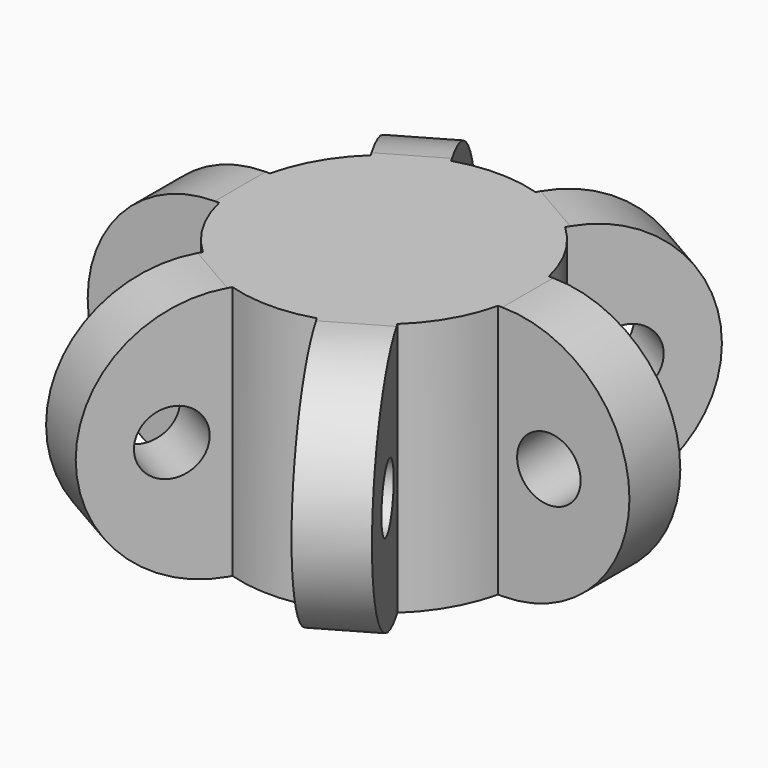
from build123d import *

# Parameters (mm, degrees)
F0_R            = 28.575
F1_DEPTH        = 50.8
F2_R            = 25.4
F3_DEPTH        = 25.4
F5_DEPTH        = 6.35
F5_DEPTH_BACK   = 6.35
F5_COPIES_COUNT = 6
F6_R            = 6.35
F7_DEPTH        = 25.4
F7_COPIES_COUNT = 6


# Not quite as in the source:
# - a pattern or mirror of a feature is missing from the dataset's text; its kind, count and spacing are read off the source's solid


with BuildPart() as f1:
    # F0 (on Top) → F1 (new body)
    with BuildSketch(Plane.XY):
        Circle(F0_R)
    extrude(amount=F1_DEPTH)

    # F2 (on face) → F3 (cut)
    with BuildSketch(Plane(origin=(0, 0, 0), x_dir=(1, 0, 0), z_dir=(0, 0, -1))):
        Circle(F2_R)
    extrude(amount=-F3_DEPTH, mode=Mode.SUBTRACT)

    # F4 (on Front) → F5 (join, two sides)
    with BuildSketch(Plane.XZ) as f5_sk:
        with BuildLine():
            ThreePointArc((-28.718591857, 50.8), (-54.118591857, 25.4), (-28.718591857, 0))
            Line((-28.718591857, 0), (-22.9244896994, 0))
            Line((-22.9244896994, 0), (-22.9244896994, 50.8))
            Line((-22.9244896994, 50.8), (-28.718591857, 50.8))
        make_face()
    f5 = extrude(amount=F5_DEPTH) + extrude(f5_sk.sketch, amount=-F5_DEPTH_BACK)

    # F5_copies: F5 ×6 about axis
    f5_copies_axis = Axis((0, 0, 0), (0, 0, 1))
    for i in range(1, F5_COPIES_COUNT):
        add(f5.rotate(f5_copies_axis, i * 360 / F5_COPIES_COUNT))

    # F6 (on face) → F7 (cut)
    with BuildSketch(Plane.XZ.offset(6.35)):
        with Locations((-38.02051193, 25.4)):
            Circle(F6_R)
    f7 = extrude(amount=-F7_DEPTH, mode=Mode.SUBTRACT)

    # F7_copies: F7 ×6 about axis
    f7_copies_axis = Axis((0, 0, 0), (0, 0, 1))
    for i in range(1, F7_COPIES_COUNT):
        add(f7.rotate(f7_copies_axis, i * 360 / F7_COPIES_COUNT), mode=Mode.SUBTRACT)


solid = f1.part
